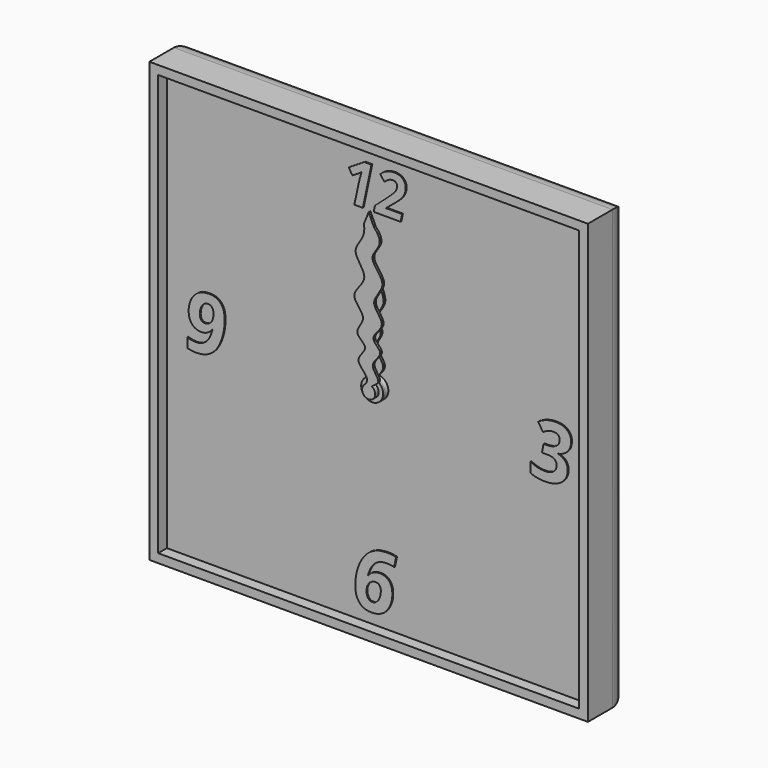
from build123d import *

# Parameters (mm, degrees)
F0_W            = 200
F0_H            = 200
F1_DEPTH        = 24
F2_R            = 10
F3_T            = -4
F4_R            = 5
F4_R_2          = 3
F5_DEPTH        = 2
F6_DEPTH        = 19
F7_DEPTH        = 8
F9_DEPTH        = 4
F11_DEPTH       = 4
F12_R           = 5
F12_R_2         = 3
F13_DEPTH       = 2
F14_R           = 3
F15_DEPTH       = 4
F17_DEPTH       = 4
F18_R           = 3
F19_DEPTH       = 2
F20_W           = 196
F20_H           = 196
F20_R           = 5
F21_DEPTH       = 1
F23_R           = 5
F23_R_2         = 3
F24_DEPTH       = 2
F25_TEXT_SIZE   = 26.048026048
F25_TEXT_SIZE_2 = 34.7222222222
F25_TEXT_SIZE_3 = 35.8387257342
F26_DEPTH       = 0.5
F27_DEPTH       = 1
F28_R           = 5
F28_R_2         = 3
F29_DEPTH       = 5
F30_R           = 3
F31_DEPTH       = 1
F33_DEPTH       = 1
F34_R           = 25
F35_DEPTH       = 10
F36_W           = 1.5
F36_H           = 6
F36_W_2         = 6
F36_H_2         = 1.5
F37_DEPTH       = 0.5
F38_R           = 3.75
F39_DEPTH       = 5
F43_DEPTH       = 1
F45_DEPTH       = 1


# Not quite as in the source:
# - Text() gives the source's letters only with a copy of the font that has no kerning and outlines rounded to 1/6400 em; it was checked with that copy


with BuildPart() as f1:
    # F0 (on Front) → F1 (new body)
    with BuildSketch(Plane.XZ):
        Rectangle(F0_W, F0_H)
    extrude(amount=F1_DEPTH)

    # F2
    f2_edges = [f1.edges().sort_by_distance(p)[0] for p in [
        (0, 0, 100),
        (-100, 0, 0),
        (0, 0, -100),
        (100, 0, 0),
    ]]
    fillet(f2_edges, radius=F2_R)

    # F3
    f3_openings = [f1.faces().sort_by_distance(p)[0] for p in [
        (0, -24, 0),
    ]]
    offset(amount=F3_T, openings=f3_openings)

    # F4 (on face) → F5 (join)
    with BuildSketch(Plane.XZ.offset(4)):
        Circle(F4_R)
        Circle(F4_R_2, mode=Mode.SUBTRACT)
        with Locations((40, 0)):
            Circle(F4_R)
        with Locations((40, 0)):
            Circle(F4_R_2, mode=Mode.SUBTRACT)
    extrude(amount=F5_DEPTH)


with BuildPart() as f6:
    # F6 (new): a face of the model
    f6_faces = [f1.part.faces().sort_by_distance(p)[0] for p in [
        (0, -4, 0),
    ]]
    extrude(f6_faces, amount=F6_DEPTH)

    # F8 (on face) → F9 (join)
    with BuildSketch(Plane.XZ.offset(6)):
        with BuildLine():
            ThreePointArc((9.2729637667, -1.3794085621), (9.3494561423, -0.6915886375), (9.375, 0))
            ThreePointArc((9.375, 0), (9.3494561423, 0.6915886375), (9.2729637667, 1.3794085621))
            ThreePointArc((9.2729637667, 1.3794085621), (8.9161548403, 2.8970343223), (8.3127812852, 4.3345463782))
            ThreePointArc((8.3127812852, 4.3345463782), (7.5845343223, 5.5104867402), (6.6911892658, 6.566476316))
            ThreePointArc((6.6911892658, 6.566476316), (5.5104867402, 7.5845343223), (4.1773988938, 8.3928519278))
            ThreePointArc((4.1773988938, 8.3928519278), (2.8970343223, 8.9161548403), (1.5536078905, 9.2453733036))
            ThreePointArc((1.5536078905, 9.2453733036), (0, 9.375), (-1.5536078905, 9.2453733036))
            ThreePointArc((-1.5536078905, 9.2453733036), (-2.8970343223, 8.9161548403), (-4.1773988938, 8.3928519278))
            ThreePointArc((-4.1773988938, 8.3928519278), (-5.5104867402, 7.5845343223), (-6.6911892658, 6.566476316))
            ThreePointArc((-6.6911892658, 6.566476316), (-7.5845343223, 5.5104867402), (-8.3127812852, 4.3345463782))
            ThreePointArc((-8.3127812852, 4.3345463782), (-8.9161548403, 2.8970343223), (-9.2729637667, 1.3794085621))
            ThreePointArc((-9.2729637667, 1.3794085621), (-9.375, 0), (-9.2729637667, -1.3794085621))
            ThreePointArc((-9.2729637667, -1.3794085621), (-8.9161548403, -2.8970343223), (-8.3127812852, -4.3345463782))
            ThreePointArc((-8.3127812852, -4.3345463782), (-7.5845343223, -5.5104867402), (-6.6911892658, -6.566476316))
            ThreePointArc((-6.6911892658, -6.566476316), (-5.5104867402, -7.5845343223), (-4.1773988938, -8.3928519278))
            ThreePointArc((-4.1773988938, -8.3928519278), (-2.8970343223, -8.9161548403), (-1.5536078905, -9.2453733036))
            ThreePointArc((-1.5536078905, -9.2453733036), (0, -9.375), (1.5536078905, -9.2453733036))
            ThreePointArc((1.5536078905, -9.2453733036), (2.8970343223, -8.9161548403), (4.1773988938, -8.3928519278))
            ThreePointArc((4.1773988938, -8.3928519278), (5.5104867402, -7.5845343223), (6.6911892658, -6.566476316))
            ThreePointArc((6.6911892658, -6.566476316), (7.5845343223, -5.5104867402), (8.3127812852, -4.3345463782))
            ThreePointArc((8.3127812852, -4.3345463782), (8.9161548403, -2.8970343223), (9.2729637667, -1.3794085621))
        make_face()
        with BuildLine():
            ThreePointArc((8.3127812852, 4.3345463782), (8.9161548403, 2.8970343223), (9.2729637667, 1.3794085621))
            Line((9.2729637667, 1.3794085621), (11.1823199426, 2.3946312492))
            Line((11.1823199426, 2.3946312492), (10.8182678729, 3.515068311))
            Line((10.8182678729, 3.515068311), (10.4542158031, 4.6355053728))
            Line((10.4542158031, 4.6355053728), (8.3127812852, 4.3345463782))
        make_face()
        with BuildLine():
            Line((11.1823199426, -2.3946312492), (9.2729637667, -1.3794085621))
            ThreePointArc((9.2729637667, -1.3794085621), (8.9161548403, -2.8970343223), (8.3127812852, -4.3345463782))
            Line((8.3127812852, -4.3345463782), (10.4542158031, -4.6355053728))
            Line((10.4542158031, -4.6355053728), (10.8182678729, -3.515068311))
            Line((10.8182678729, -3.515068311), (11.1823199426, -2.3946312492))
        make_face()
        with BuildLine():
            ThreePointArc((4.1773988938, 8.3928519278), (5.5104867402, 7.5845343223), (6.6911892658, 6.566476316))
            Line((6.6911892658, 6.566476316), (7.6391579371, 8.5101001246))
            Line((7.6391579371, 8.5101001246), (6.6860572448, 9.202568311))
            Line((6.6860572448, 9.202568311), (5.7329565525, 9.8950364974))
            Line((5.7329565525, 9.8950364974), (4.1773988938, 8.3928519278))
        make_face()
        with BuildLine():
            Line((7.6391579371, -8.5101001246), (6.6911892658, -6.566476316))
            ThreePointArc((6.6911892658, -6.566476316), (5.5104867402, -7.5845343223), (4.1773988938, -8.3928519278))
            Line((4.1773988938, -8.3928519278), (5.7329565525, -9.8950364974))
            Line((5.7329565525, -9.8950364974), (6.6860572448, -9.202568311))
            Line((6.6860572448, -9.202568311), (7.6391579371, -8.5101001246))
        make_face()
        with BuildLine():
            ThreePointArc((-1.5536078905, 9.2453733036), (0, 9.375), (1.5536078905, 9.2453733036))
            Line((1.5536078905, 9.2453733036), (1.1780972451, 11.375))
            Line((1.1780972451, 11.375), (0, 11.375))
            Line((0, 11.375), (-1.1780972451, 11.375))
            Line((-1.1780972451, 11.375), (-1.5536078905, 9.2453733036))
        make_face()
        with BuildLine():
            Line((1.1780972451, -11.375), (1.5536078905, -9.2453733036))
            ThreePointArc((1.5536078905, -9.2453733036), (0, -9.375), (-1.5536078905, -9.2453733036))
            Line((-1.5536078905, -9.2453733036), (-1.1780972451, -11.375))
            Line((-1.1780972451, -11.375), (0, -11.375))
            Line((0, -11.375), (1.1780972451, -11.375))
        make_face()
        with BuildLine():
            ThreePointArc((-6.6911892658, 6.566476316), (-5.5104867402, 7.5845343223), (-4.1773988938, 8.3928519278))
            Line((-4.1773988938, 8.3928519278), (-5.7329565525, 9.8950364974))
            Line((-5.7329565525, 9.8950364974), (-6.6860572448, 9.202568311))
            Line((-6.6860572448, 9.202568311), (-7.6391579371, 8.5101001246))
            Line((-7.6391579371, 8.5101001246), (-6.6911892658, 6.566476316))
        make_face()
        with BuildLine():
            Line((-5.7329565525, -9.8950364974), (-4.1773988938, -8.3928519278))
            ThreePointArc((-4.1773988938, -8.3928519278), (-5.5104867402, -7.5845343223), (-6.6911892658, -6.566476316))
            Line((-6.6911892658, -6.566476316), (-7.6391579371, -8.5101001246))
            Line((-7.6391579371, -8.5101001246), (-6.6860572448, -9.202568311))
            Line((-6.6860572448, -9.202568311), (-5.7329565525, -9.8950364974))
        make_face()
        with BuildLine():
            ThreePointArc((-9.2729637667, 1.3794085621), (-8.9161548403, 2.8970343223), (-8.3127812852, 4.3345463782))
            Line((-8.3127812852, 4.3345463782), (-10.4542158031, 4.6355053728))
            Line((-10.4542158031, 4.6355053728), (-10.8182678729, 3.515068311))
            Line((-10.8182678729, 3.515068311), (-11.1823199426, 2.3946312492))
            Line((-11.1823199426, 2.3946312492), (-9.2729637667, 1.3794085621))
        make_face()
        with BuildLine():
            Line((-10.4542158031, -4.6355053728), (-8.3127812852, -4.3345463782))
            ThreePointArc((-8.3127812852, -4.3345463782), (-8.9161548403, -2.8970343223), (-9.2729637667, -1.3794085621))
            Line((-9.2729637667, -1.3794085621), (-11.1823199426, -2.3946312492))
            Line((-11.1823199426, -2.3946312492), (-10.8182678729, -3.515068311))
            Line((-10.8182678729, -3.515068311), (-10.4542158031, -4.6355053728))
        make_face()
    extrude(amount=F9_DEPTH)

    # F32 (on face) → F33 (join)
    with BuildSketch(Plane.XZ.offset(23)):
        with BuildLine():
            ThreePointArc((-1.4071694433, 2.6495045118), (-1.5457185498, -2.5711386903), (3, 0))
            ThreePointArc((3, 0), (2.5711386903, 1.5457185498), (1.4071694433, 2.6495045118))
            ThreePointArc((1.4071694433, 2.6495045118), (0, 3), (-1.4071694433, 2.6495045118))
        make_face()
        with BuildLine():
            ThreePointArc((-1.4071694433, 2.6495045118), (0, 3), (1.4071694433, 2.6495045118))
            add(Edge.make_bspline(
                [(1.4071694433, 2.6495045118), (3.0296074566, 3.8772159389), (6.3039386169, 5.5103249168), (-0.9360700478, 11.6043913935), (8.3069373895, 17.3298364556), (-1.1275149054, 22.1266315872), (9.6827878452, 28.9044203262), (-1.2541438892, 36.5685190657), (10.3089623501, 45.1730816435), (-1.6342219672, 53.9788895131), (6.9529120063, 60.5380152538), (4.0439217419, 65.1597511734), (2.5257738307, 66.6606426239)],
                knots=[0, 0, 0, 0, 0.0782288026, 0.1704201684, 0.2679376052, 0.3576739035, 0.4617977775, 0.5704836043, 0.6853974221, 0.803568051, 0.9061859038, 1, 1, 1, 1], degree=3))
            Line((2.5257738307, 66.6606426239), (0, 72.1388086677))
            Line((0, 72.1388086677), (-2.1966320928, 66.6606426239))
            add(Edge.make_bspline(
                [(-1.4071694433, 2.6495045118), (-0.8303886963, 3.6654317675), (0.0856435734, 6.0391183116), (-7.5716818535, 11.2944408044), (1.3992736808, 17.5147965731), (-8.220861358, 21.8793846794), (0.7776188709, 29.1436053021), (-10.5454136086, 36.5799618446), (2.0038158577, 45.007894694), (-8.7780353011, 54.0426044509), (-2.1019578832, 60.4375853407), (-1.7889988447, 65.0866098847), (-2.1966320928, 66.6606426239)],
                knots=[0, 0, 0, 0, 0.0669744584, 0.165033993, 0.2625239648, 0.3553389335, 0.4570466298, 0.5683341016, 0.6867000587, 0.8048964881, 0.908333357, 1, 1, 1, 1], degree=3))
        make_face()
    extrude(amount=F33_DEPTH)


with BuildPart() as f7:
    # F7 (new): a face of the model
    f7_faces = [f1.part.faces().sort_by_distance(p)[0] for p in [
        (40, -4, 0),
    ]]
    extrude(f7_faces, amount=F7_DEPTH)

    # F10 (on face) → F11 (join)
    with BuildSketch(Plane.XZ.offset(6)):
        with BuildLine():
            ThreePointArc((68.0829066802, -1.5381733945), (68.1144747006, -0.7693746225), (68.125, 0))
            ThreePointArc((68.125, 0), (68.1144747006, 0.7693746225), (68.0829066802, 1.5381733945))
            ThreePointArc((68.0829066802, 1.5381733945), (67.9709283072, 2.9398630294), (67.7890320221, 4.3342039956))
            ThreePointArc((67.7890320221, 4.3342039956), (67.5104012706, 5.8475163042), (67.1494235596, 7.3433252263))
            ThreePointArc((67.1494235596, 7.3433252263), (66.7484645208, 8.6911029668), (66.280643318, 10.0171558733))
            ThreePointArc((66.280643318, 10.0171558733), (65.6934659962, 11.4394680865), (65.0293803521, 12.8275385085))
            ThreePointArc((65.0293803521, 12.8275385085), (64.3569644814, 14.0625), (63.6236643925, 15.2623099717))
            ThreePointArc((63.6236643925, 15.2623099717), (62.7536029668, 16.5314602207), (61.815433119, 17.7511268046))
            ThreePointArc((61.815433119, 17.7511268046), (60.9009482166, 18.8192983038), (59.934217974, 19.8404278876))
            ThreePointArc((59.934217974, 19.8404278876), (58.8192983038, 20.9009482166), (57.6480467764, 21.8989056799))
            ThreePointArc((57.6480467764, 21.8989056799), (56.5314602207, 22.7536029668), (55.3735505752, 23.5514238999))
            ThreePointArc((55.3735505752, 23.5514238999), (54.0625, 24.3569644814), (52.709356105, 25.0895972944))
            ThreePointArc((52.709356105, 25.0895972944), (51.4394680865, 25.6934659962), (50.1409852457, 26.2331096755))
            ThreePointArc((50.1409852457, 26.2331096755), (48.6911029668, 26.7484645208), (47.2152055856, 27.1837531139))
            ThreePointArc((47.2152055856, 27.1837531139), (45.8475163042, 27.5104012706), (44.4652101991, 27.7682826779))
            ThreePointArc((44.4652101991, 27.7682826779), (42.9398630294, 27.9709283072), (41.4057159597, 28.0898484802))
            ThreePointArc((41.4057159597, 28.0898484802), (40, 28.125), (38.5942840403, 28.0898484802))
            ThreePointArc((38.5942840403, 28.0898484802), (37.0601369706, 27.9709283072), (35.5347898009, 27.7682826779))
            ThreePointArc((35.5347898009, 27.7682826779), (34.1524836958, 27.5104012706), (32.7847944144, 27.1837531139))
            ThreePointArc((32.7847944144, 27.1837531139), (31.3088970332, 26.7484645208), (29.8590147543, 26.2331096755))
            ThreePointArc((29.8590147543, 26.2331096755), (28.5605319135, 25.6934659962), (27.290643895, 25.0895972944))
            ThreePointArc((27.290643895, 25.0895972944), (25.9375, 24.3569644814), (24.6264494248, 23.5514238999))
            ThreePointArc((24.6264494248, 23.5514238999), (23.4685397793, 22.7536029668), (22.3519532236, 21.8989056799))
            ThreePointArc((22.3519532236, 21.8989056799), (21.1807016962, 20.9009482166), (20.065782026, 19.8404278876))
            ThreePointArc((20.065782026, 19.8404278876), (19.0990517834, 18.8192983038), (18.184566881, 17.7511268046))
            ThreePointArc((18.184566881, 17.7511268046), (17.2463970332, 16.5314602207), (16.3763356075, 15.2623099717))
            ThreePointArc((16.3763356075, 15.2623099717), (15.6430355186, 14.0625), (14.9706196479, 12.8275385085))
            ThreePointArc((14.9706196479, 12.8275385085), (14.3065340038, 11.4394680865), (13.719356682, 10.0171558733))
            ThreePointArc((13.719356682, 10.0171558733), (13.2515354792, 8.6911029668), (12.8505764404, 7.3433252263))
            ThreePointArc((12.8505764404, 7.3433252263), (12.4895987294, 5.8475163042), (12.2109679779, 4.3342039956))
            ThreePointArc((12.2109679779, 4.3342039956), (12.0290716928, 2.9398630294), (11.9170933198, 1.5381733945))
            ThreePointArc((11.9170933198, 1.5381733945), (11.875, 0), (11.9170933198, -1.5381733945))
            ThreePointArc((11.9170933198, -1.5381733945), (12.0290716928, -2.9398630294), (12.2109679779, -4.3342039956))
            ThreePointArc((12.2109679779, -4.3342039956), (12.4895987294, -5.8475163042), (12.8505764404, -7.3433252263))
            ThreePointArc((12.8505764404, -7.3433252263), (13.2515354792, -8.6911029668), (13.719356682, -10.0171558733))
            ThreePointArc((13.719356682, -10.0171558733), (14.3065340038, -11.4394680865), (14.9706196479, -12.8275385085))
            ThreePointArc((14.9706196479, -12.8275385085), (15.6430355186, -14.0625), (16.3763356075, -15.2623099717))
            ThreePointArc((16.3763356075, -15.2623099717), (17.2463970332, -16.5314602207), (18.184566881, -17.7511268046))
            ThreePointArc((18.184566881, -17.7511268046), (19.0990517834, -18.8192983038), (20.065782026, -19.8404278876))
            ThreePointArc((20.065782026, -19.8404278876), (21.1807016962, -20.9009482166), (22.3519532236, -21.8989056799))
            ThreePointArc((22.3519532236, -21.8989056799), (23.4685397793, -22.7536029668), (24.6264494248, -23.5514238999))
            ThreePointArc((24.6264494248, -23.5514238999), (25.9375, -24.3569644814), (27.290643895, -25.0895972944))
            ThreePointArc((27.290643895, -25.0895972944), (28.5605319135, -25.6934659962), (29.8590147543, -26.2331096755))
            ThreePointArc((29.8590147543, -26.2331096755), (31.3088970332, -26.7484645208), (32.7847944144, -27.1837531139))
            ThreePointArc((32.7847944144, -27.1837531139), (34.1524836958, -27.5104012706), (35.5347898009, -27.7682826779))
            ThreePointArc((35.5347898009, -27.7682826779), (37.0601369706, -27.9709283072), (38.5942840403, -28.0898484802))
            ThreePointArc((38.5942840403, -28.0898484802), (40, -28.125), (41.4057159597, -28.0898484802))
            ThreePointArc((41.4057159597, -28.0898484802), (42.9398630294, -27.9709283072), (44.4652101991, -27.7682826779))
            ThreePointArc((44.4652101991, -27.7682826779), (45.8475163042, -27.5104012706), (47.2152055856, -27.1837531139))
            ThreePointArc((47.2152055856, -27.1837531139), (48.6911029668, -26.7484645208), (50.1409852457, -26.2331096755))
            ThreePointArc((50.1409852457, -26.2331096755), (51.4394680865, -25.6934659962), (52.709356105, -25.0895972944))
            ThreePointArc((52.709356105, -25.0895972944), (54.0625, -24.3569644814), (55.3735505752, -23.5514238999))
            ThreePointArc((55.3735505752, -23.5514238999), (56.5314602207, -22.7536029668), (57.6480467764, -21.8989056799))
            ThreePointArc((57.6480467764, -21.8989056799), (58.8192983038, -20.9009482166), (59.934217974, -19.8404278876))
            ThreePointArc((59.934217974, -19.8404278876), (60.9009482166, -18.8192983038), (61.815433119, -17.7511268046))
            ThreePointArc((61.815433119, -17.7511268046), (62.7536029668, -16.5314602207), (63.6236643925, -15.2623099717))
            ThreePointArc((63.6236643925, -15.2623099717), (64.3569644814, -14.0625), (65.0293803521, -12.8275385085))
            ThreePointArc((65.0293803521, -12.8275385085), (65.6934659962, -11.4394680865), (66.280643318, -10.0171558733))
            ThreePointArc((66.280643318, -10.0171558733), (66.7484645208, -8.6911029668), (67.1494235596, -7.3433252263))
            ThreePointArc((67.1494235596, -7.3433252263), (67.5104012706, -5.8475163042), (67.7890320221, -4.3342039956))
            ThreePointArc((67.7890320221, -4.3342039956), (67.9709283072, -2.9398630294), (68.0829066802, -1.5381733945))
        make_face()
        with BuildLine():
            ThreePointArc((68.0829066802, 1.5381733945), (68.1144747006, 0.7693746225), (68.125, 0))
            ThreePointArc((68.125, 0), (68.1144747006, -0.7693746225), (68.0829066802, -1.5381733945))
            Line((68.0829066802, -1.5381733945), (70.125, -1.1780972451))
            Line((70.125, -1.1780972451), (70.125, 0))
            Line((70.125, 0), (70.125, 1.1780972451))
            Line((70.125, 1.1780972451), (68.0829066802, 1.5381733945))
        make_face()
        with BuildLine():
            ThreePointArc((67.1494235596, 7.3433252263), (67.5104012706, 5.8475163042), (67.7890320221, 4.3342039956))
            Line((67.7890320221, 4.3342039956), (69.7116366623, 5.1109866922))
            Line((69.7116366623, 5.1109866922), (69.4666964721, 6.2633396859))
            Line((69.4666964721, 6.2633396859), (69.2217562819, 7.4156926796))
            Line((69.2217562819, 7.4156926796), (67.1494235596, 7.3433252263))
        make_face()
        with BuildLine():
            Line((69.7116366623, -5.1109866922), (67.7890320221, -4.3342039956))
            ThreePointArc((67.7890320221, -4.3342039956), (67.5104012706, -5.8475163042), (67.1494235596, -7.3433252263))
            Line((67.1494235596, -7.3433252263), (69.2217562819, -7.4156926796))
            Line((69.2217562819, -7.4156926796), (69.4666964721, -6.2633396859))
            Line((69.4666964721, -6.2633396859), (69.7116366623, -5.1109866922))
        make_face()
        with BuildLine():
            ThreePointArc((65.0293803521, 12.8275385085), (65.6934659962, 11.4394680865), (66.280643318, 10.0171558733))
            Line((66.280643318, 10.0171558733), (67.9997322302, 11.1766959857))
            Line((67.9997322302, 11.1766959857), (67.5205569115, 12.2529413727))
            Line((67.5205569115, 12.2529413727), (67.0413815928, 13.3291867596))
            Line((67.0413815928, 13.3291867596), (65.0293803521, 12.8275385085))
        make_face()
        with BuildLine():
            Line((67.9997322302, -11.1766959857), (66.280643318, -10.0171558733))
            ThreePointArc((66.280643318, -10.0171558733), (65.6934659962, -11.4394680865), (65.0293803521, -12.8275385085))
            Line((65.0293803521, -12.8275385085), (67.0413815928, -13.3291867596))
            Line((67.0413815928, -13.3291867596), (67.5205569115, -12.2529413727))
            Line((67.5205569115, -12.2529413727), (67.9997322302, -11.1766959857))
        make_face()
        with BuildLine():
            ThreePointArc((61.815433119, 17.7511268046), (62.7536029668, 16.5314602207), (63.6236643925, 15.2623099717))
            Line((63.6236643925, 15.2623099717), (65.064105142, 16.753930033))
            Line((65.064105142, 16.753930033), (64.3716369555, 17.7070307253))
            Line((64.3716369555, 17.7070307253), (63.6791687691, 18.6601314176))
            Line((63.6791687691, 18.6601314176), (61.815433119, 17.7511268046))
        make_face()
        with BuildLine():
            Line((65.064105142, -16.753930033), (63.6236643925, -15.2623099717))
            ThreePointArc((63.6236643925, -15.2623099717), (62.7536029668, -16.5314602207), (61.815433119, -17.7511268046))
            Line((61.815433119, -17.7511268046), (63.6791687691, -18.6601314176))
            Line((63.6791687691, -18.6601314176), (64.3716369555, -17.7070307253))
            Line((64.3716369555, -17.7070307253), (65.064105142, -16.753930033))
        make_face()
        with BuildLine():
            ThreePointArc((57.6480467764, 21.8989056799), (58.8192983038, 20.9009482166), (59.934217974, 19.8404278876))
            Line((59.934217974, 19.8404278876), (61.0330563882, 21.5989369435))
            Line((61.0330563882, 21.5989369435), (60.1575595166, 22.3872378675))
            Line((60.1575595166, 22.3872378675), (59.282062645, 23.1755387915))
            Line((59.282062645, 23.1755387915), (57.6480467764, 21.8989056799))
        make_face()
        with BuildLine():
            Line((61.0330563882, -21.5989369435), (59.934217974, -19.8404278876))
            ThreePointArc((59.934217974, -19.8404278876), (58.8192983038, -20.9009482166), (57.6480467764, -21.8989056799))
            Line((57.6480467764, -21.8989056799), (59.282062645, -23.1755387915))
            Line((59.282062645, -23.1755387915), (60.1575595166, -22.3872378675))
            Line((60.1575595166, -22.3872378675), (61.0330563882, -21.5989369435))
        make_face()
        with BuildLine():
            ThreePointArc((52.709356105, 25.0895972944), (54.0625, 24.3569644814), (55.3735505752, 23.5514238999))
            Line((55.3735505752, 23.5514238999), (56.0827621424, 25.4999666665))
            Line((56.0827621424, 25.4999666665), (55.0625, 26.089015289))
            Line((55.0625, 26.089015289), (54.0422378576, 26.6780639116))
            Line((54.0422378576, 26.6780639116), (52.709356105, 25.0895972944))
        make_face()
        with BuildLine():
            Line((56.0827621424, -25.4999666665), (55.3735505752, -23.5514238999))
            ThreePointArc((55.3735505752, -23.5514238999), (54.0625, -24.3569644814), (52.709356105, -25.0895972944))
            Line((52.709356105, -25.0895972944), (54.0422378576, -26.6780639116))
            Line((54.0422378576, -26.6780639116), (55.0625, -26.089015289))
            Line((55.0625, -26.089015289), (56.0827621424, -25.4999666665))
        make_face()
        with BuildLine():
            ThreePointArc((47.2152055856, 27.1837531139), (48.6911029668, 26.7484645208), (50.1409852457, 26.2331096755))
            Line((50.1409852457, 26.2331096755), (50.4295740173, 28.2865254836))
            Line((50.4295740173, 28.2865254836), (49.3091369555, 28.6505775534))
            Line((49.3091369555, 28.6505775534), (48.1886998938, 29.0146296232))
            Line((48.1886998938, 29.0146296232), (47.2152055856, 27.1837531139))
        make_face()
        with BuildLine():
            Line((50.4295740173, -28.2865254836), (50.1409852457, -26.2331096755))
            ThreePointArc((50.1409852457, -26.2331096755), (48.6911029668, -26.7484645208), (47.2152055856, -27.1837531139))
            Line((47.2152055856, -27.1837531139), (48.1886998938, -29.0146296232))
            Line((48.1886998938, -29.0146296232), (49.3091369555, -28.6505775534))
            Line((49.3091369555, -28.6505775534), (50.4295740173, -28.2865254836))
        make_face()
        with BuildLine():
            ThreePointArc((41.4057159597, 28.0898484802), (42.9398630294, 27.9709283072), (44.4652101991, 27.7682826779))
            Line((44.4652101991, 27.7682826779), (44.3205634611, 29.8368274034))
            Line((44.3205634611, 29.8368274034), (43.1489199559, 29.959972098))
            Line((43.1489199559, 29.959972098), (41.9772764508, 30.0831167926))
            Line((41.9772764508, 30.0831167926), (41.4057159597, 28.0898484802))
        make_face()
        with BuildLine():
            Line((44.3205634611, -29.8368274034), (44.4652101991, -27.7682826779))
            ThreePointArc((44.4652101991, -27.7682826779), (42.9398630294, -27.9709283072), (41.4057159597, -28.0898484802))
            Line((41.4057159597, -28.0898484802), (41.9772764508, -30.0831167926))
            Line((41.9772764508, -30.0831167926), (43.1489199559, -29.959972098))
            Line((43.1489199559, -29.959972098), (44.3205634611, -29.8368274034))
        make_face()
        with BuildLine():
            ThreePointArc((35.5347898009, 27.7682826779), (37.0601369706, 27.9709283072), (38.5942840403, 28.0898484802))
            Line((38.5942840403, 28.0898484802), (38.0227235492, 30.0831167926))
            Line((38.0227235492, 30.0831167926), (36.8510800441, 29.959972098))
            Line((36.8510800441, 29.959972098), (35.6794365389, 29.8368274034))
            Line((35.6794365389, 29.8368274034), (35.5347898009, 27.7682826779))
        make_face()
        with BuildLine():
            Line((38.0227235492, -30.0831167926), (38.5942840403, -28.0898484802))
            ThreePointArc((38.5942840403, -28.0898484802), (37.0601369706, -27.9709283072), (35.5347898009, -27.7682826779))
            Line((35.5347898009, -27.7682826779), (35.6794365389, -29.8368274034))
            Line((35.6794365389, -29.8368274034), (36.8510800441, -29.959972098))
            Line((36.8510800441, -29.959972098), (38.0227235492, -30.0831167926))
        make_face()
        with BuildLine():
            ThreePointArc((29.8590147543, 26.2331096755), (31.3088970332, 26.7484645208), (32.7847944144, 27.1837531139))
            Line((32.7847944144, 27.1837531139), (31.8113001062, 29.0146296232))
            Line((31.8113001062, 29.0146296232), (30.6908630445, 28.6505775534))
            Line((30.6908630445, 28.6505775534), (29.5704259827, 28.2865254836))
            Line((29.5704259827, 28.2865254836), (29.8590147543, 26.2331096755))
        make_face()
        with BuildLine():
            Line((31.8113001062, -29.0146296232), (32.7847944144, -27.1837531139))
            ThreePointArc((32.7847944144, -27.1837531139), (31.3088970332, -26.7484645208), (29.8590147543, -26.2331096755))
            Line((29.8590147543, -26.2331096755), (29.5704259827, -28.2865254836))
            Line((29.5704259827, -28.2865254836), (30.6908630445, -28.6505775534))
            Line((30.6908630445, -28.6505775534), (31.8113001062, -29.0146296232))
        make_face()
        with BuildLine():
            ThreePointArc((24.6264494248, 23.5514238999), (25.9375, 24.3569644814), (27.290643895, 25.0895972944))
            Line((27.290643895, 25.0895972944), (25.9577621424, 26.6780639116))
            Line((25.9577621424, 26.6780639116), (24.9375, 26.089015289))
            Line((24.9375, 26.089015289), (23.9172378576, 25.4999666665))
            Line((23.9172378576, 25.4999666665), (24.6264494248, 23.5514238999))
        make_face()
        with BuildLine():
            Line((25.9577621424, -26.6780639116), (27.290643895, -25.0895972944))
            ThreePointArc((27.290643895, -25.0895972944), (25.9375, -24.3569644814), (24.6264494248, -23.5514238999))
            Line((24.6264494248, -23.5514238999), (23.9172378576, -25.4999666665))
            Line((23.9172378576, -25.4999666665), (24.9375, -26.089015289))
            Line((24.9375, -26.089015289), (25.9577621424, -26.6780639116))
        make_face()
        with BuildLine():
            ThreePointArc((20.065782026, 19.8404278876), (21.1807016962, 20.9009482166), (22.3519532236, 21.8989056799))
            Line((22.3519532236, 21.8989056799), (20.717937355, 23.1755387915))
            Line((20.717937355, 23.1755387915), (19.8424404834, 22.3872378675))
            Line((19.8424404834, 22.3872378675), (18.9669436118, 21.5989369435))
            Line((18.9669436118, 21.5989369435), (20.065782026, 19.8404278876))
        make_face()
        with BuildLine():
            Line((20.717937355, -23.1755387915), (22.3519532236, -21.8989056799))
            ThreePointArc((22.3519532236, -21.8989056799), (21.1807016962, -20.9009482166), (20.065782026, -19.8404278876))
            Line((20.065782026, -19.8404278876), (18.9669436118, -21.5989369435))
            Line((18.9669436118, -21.5989369435), (19.8424404834, -22.3872378675))
            Line((19.8424404834, -22.3872378675), (20.717937355, -23.1755387915))
        make_face()
        with BuildLine():
            ThreePointArc((16.3763356075, 15.2623099717), (17.2463970332, 16.5314602207), (18.184566881, 17.7511268046))
            Line((18.184566881, 17.7511268046), (16.3208312309, 18.6601314176))
            Line((16.3208312309, 18.6601314176), (15.6283630445, 17.7070307253))
            Line((15.6283630445, 17.7070307253), (14.935894858, 16.753930033))
            Line((14.935894858, 16.753930033), (16.3763356075, 15.2623099717))
        make_face()
        with BuildLine():
            Line((16.3208312309, -18.6601314176), (18.184566881, -17.7511268046))
            ThreePointArc((18.184566881, -17.7511268046), (17.2463970332, -16.5314602207), (16.3763356075, -15.2623099717))
            Line((16.3763356075, -15.2623099717), (14.935894858, -16.753930033))
            Line((14.935894858, -16.753930033), (15.6283630445, -17.7070307253))
            Line((15.6283630445, -17.7070307253), (16.3208312309, -18.6601314176))
        make_face()
        with BuildLine():
            ThreePointArc((13.719356682, 10.0171558733), (14.3065340038, 11.4394680865), (14.9706196479, 12.8275385085))
            Line((14.9706196479, 12.8275385085), (12.9586184072, 13.3291867596))
            Line((12.9586184072, 13.3291867596), (12.4794430885, 12.2529413727))
            Line((12.4794430885, 12.2529413727), (12.0002677698, 11.1766959857))
            Line((12.0002677698, 11.1766959857), (13.719356682, 10.0171558733))
        make_face()
        with BuildLine():
            Line((12.9586184072, -13.3291867596), (14.9706196479, -12.8275385085))
            ThreePointArc((14.9706196479, -12.8275385085), (14.3065340038, -11.4394680865), (13.719356682, -10.0171558733))
            Line((13.719356682, -10.0171558733), (12.0002677698, -11.1766959857))
            Line((12.0002677698, -11.1766959857), (12.4794430885, -12.2529413727))
            Line((12.4794430885, -12.2529413727), (12.9586184072, -13.3291867596))
        make_face()
        with BuildLine():
            ThreePointArc((12.2109679779, 4.3342039956), (12.4895987294, 5.8475163042), (12.8505764404, 7.3433252263))
            Line((12.8505764404, 7.3433252263), (10.7782437181, 7.4156926796))
            Line((10.7782437181, 7.4156926796), (10.5333035279, 6.2633396859))
            Line((10.5333035279, 6.2633396859), (10.2883633377, 5.1109866922))
            Line((10.2883633377, 5.1109866922), (12.2109679779, 4.3342039956))
        make_face()
        with BuildLine():
            Line((10.7782437181, -7.4156926796), (12.8505764404, -7.3433252263))
            ThreePointArc((12.8505764404, -7.3433252263), (12.4895987294, -5.8475163042), (12.2109679779, -4.3342039956))
            Line((12.2109679779, -4.3342039956), (10.2883633377, -5.1109866922))
            Line((10.2883633377, -5.1109866922), (10.5333035279, -6.2633396859))
            Line((10.5333035279, -6.2633396859), (10.7782437181, -7.4156926796))
        make_face()
        with BuildLine():
            ThreePointArc((11.9170933198, -1.5381733945), (11.875, 0), (11.9170933198, 1.5381733945))
            Line((11.9170933198, 1.5381733945), (9.875, 1.1780972451))
            Line((9.875, 1.1780972451), (9.875, 0))
            Line((9.875, 0), (9.875, -1.1780972451))
            Line((9.875, -1.1780972451), (11.9170933198, -1.5381733945))
        make_face()
    extrude(amount=F11_DEPTH)

    # F16 (on face) → F17 (join)
    with BuildSketch(Plane.XZ.offset(12)):
        with BuildLine():
            ThreePointArc((47.4288750323, -1.0304444454), (47.4821976298, -0.5164480894), (47.5, 0))
            ThreePointArc((47.5, 0), (47.4821976298, 0.5164480894), (47.4288750323, 1.0304444454))
            ThreePointArc((47.4288750323, 1.0304444454), (47.1329238722, 2.3176274578), (46.6157661985, 3.532936117))
            ThreePointArc((46.6157661985, 3.532936117), (46.0676274578, 4.4083893922), (45.4044061018, 5.2002302532))
            ThreePointArc((45.4044061018, 5.2002302532), (44.4083893922, 6.0676274578), (43.2756595386, 6.7468551628))
            ThreePointArc((43.2756595386, 6.7468551628), (42.3176274578, 7.1329238722), (41.3156377295, 7.3837048536))
            ThreePointArc((41.3156377295, 7.3837048536), (40, 7.5), (38.6843622705, 7.3837048536))
            ThreePointArc((38.6843622705, 7.3837048536), (37.6823725422, 7.1329238722), (36.7243404614, 6.7468551628))
            ThreePointArc((36.7243404614, 6.7468551628), (35.5916106078, 6.0676274578), (34.5955938982, 5.2002302532))
            ThreePointArc((34.5955938982, 5.2002302532), (33.9323725422, 4.4083893922), (33.3842338015, 3.532936117))
            ThreePointArc((33.3842338015, 3.532936117), (32.8670761278, 2.3176274578), (32.5711249677, 1.0304444454))
            ThreePointArc((32.5711249677, 1.0304444454), (32.5, 0), (32.5711249677, -1.0304444454))
            ThreePointArc((32.5711249677, -1.0304444454), (32.8670761278, -2.3176274578), (33.3842338015, -3.532936117))
            ThreePointArc((33.3842338015, -3.532936117), (33.9323725422, -4.4083893922), (34.5955938982, -5.2002302532))
            ThreePointArc((34.5955938982, -5.2002302532), (35.5916106078, -6.0676274578), (36.7243404614, -6.7468551628))
            ThreePointArc((36.7243404614, -6.7468551628), (37.6823725422, -7.1329238722), (38.6843622705, -7.3837048536))
            ThreePointArc((38.6843622705, -7.3837048536), (40, -7.5), (41.3156377295, -7.3837048536))
            ThreePointArc((41.3156377295, -7.3837048536), (42.3176274578, -7.1329238722), (43.2756595386, -6.7468551628))
            ThreePointArc((43.2756595386, -6.7468551628), (44.4083893922, -6.0676274578), (45.4044061018, -5.2002302532))
            ThreePointArc((45.4044061018, -5.2002302532), (46.0676274578, -4.4083893922), (46.6157661985, -3.532936117))
            ThreePointArc((46.6157661985, -3.532936117), (47.1329238722, -2.3176274578), (47.4288750323, -1.0304444454))
        make_face()
        with BuildLine():
            ThreePointArc((46.6157661985, 3.532936117), (47.1329238722, 2.3176274578), (47.4288750323, 1.0304444454))
            Line((47.4288750323, 1.0304444454), (49.3262785606, 2.0393117971))
            Line((49.3262785606, 2.0393117971), (48.743795249, 3.832011096))
            Line((48.743795249, 3.832011096), (46.6157661985, 3.532936117))
        make_face()
        with BuildLine():
            Line((49.3262785606, -2.0393117971), (47.4288750323, -1.0304444454))
            ThreePointArc((47.4288750323, -1.0304444454), (47.1329238722, -2.3176274578), (46.6157661985, -3.532936117))
            Line((46.6157661985, -3.532936117), (48.743795249, -3.832011096))
            Line((48.743795249, -3.832011096), (49.3262785606, -2.0393117971))
        make_face()
        with BuildLine():
            ThreePointArc((43.2756595386, 6.7468551628), (44.4083893922, 6.0676274578), (45.4044061018, 5.2002302532))
            Line((45.4044061018, 5.2002302532), (46.3464404506, 7.1316868974))
            Line((46.3464404506, 7.1316868974), (44.8214793429, 8.2396359957))
            Line((44.8214793429, 8.2396359957), (43.2756595386, 6.7468551628))
        make_face()
        with BuildLine():
            Line((46.3464404506, -7.1316868974), (45.4044061018, -5.2002302532))
            ThreePointArc((45.4044061018, -5.2002302532), (44.4083893922, -6.0676274578), (43.2756595386, -6.7468551628))
            Line((43.2756595386, -6.7468551628), (44.8214793429, -8.2396359957))
            Line((44.8214793429, -8.2396359957), (46.3464404506, -7.1316868974))
        make_face()
        with BuildLine():
            ThreePointArc((38.6843622705, 7.3837048536), (40, 7.5), (41.3156377295, 7.3837048536))
            Line((41.3156377295, 7.3837048536), (40.9424777961, 9.5))
            Line((40.9424777961, 9.5), (39.0575222039, 9.5))
            Line((39.0575222039, 9.5), (38.6843622705, 7.3837048536))
        make_face()
        with BuildLine():
            Line((40.9424777961, -9.5), (41.3156377295, -7.3837048536))
            ThreePointArc((41.3156377295, -7.3837048536), (40, -7.5), (38.6843622705, -7.3837048536))
            Line((38.6843622705, -7.3837048536), (39.0575222039, -9.5))
            Line((39.0575222039, -9.5), (40.9424777961, -9.5))
        make_face()
        with BuildLine():
            ThreePointArc((34.5955938982, 5.2002302532), (35.5916106078, 6.0676274578), (36.7243404614, 6.7468551628))
            Line((36.7243404614, 6.7468551628), (35.1785206571, 8.2396359957))
            Line((35.1785206571, 8.2396359957), (33.6535595494, 7.1316868974))
            Line((33.6535595494, 7.1316868974), (34.5955938982, 5.2002302532))
        make_face()
        with BuildLine():
            Line((35.1785206571, -8.2396359957), (36.7243404614, -6.7468551628))
            ThreePointArc((36.7243404614, -6.7468551628), (35.5916106078, -6.0676274578), (34.5955938982, -5.2002302532))
            Line((34.5955938982, -5.2002302532), (33.6535595494, -7.1316868974))
            Line((33.6535595494, -7.1316868974), (35.1785206571, -8.2396359957))
        make_face()
        with BuildLine():
            ThreePointArc((32.5711249677, 1.0304444454), (32.8670761278, 2.3176274578), (33.3842338015, 3.532936117))
            Line((33.3842338015, 3.532936117), (31.256204751, 3.832011096))
            Line((31.256204751, 3.832011096), (30.6737214394, 2.0393117971))
            Line((30.6737214394, 2.0393117971), (32.5711249677, 1.0304444454))
        make_face()
        with BuildLine():
            Line((31.256204751, -3.832011096), (33.3842338015, -3.532936117))
            ThreePointArc((33.3842338015, -3.532936117), (32.8670761278, -2.3176274578), (32.5711249677, -1.0304444454))
            Line((32.5711249677, -1.0304444454), (30.6737214394, -2.0393117971))
            Line((30.6737214394, -2.0393117971), (31.256204751, -3.832011096))
        make_face()
    extrude(amount=F17_DEPTH)

    # F18 (on face) → F19 (join)
    with BuildSketch(Plane.XZ.offset(16)):
        with Locations((40, 0)):
            Circle(F18_R)
    extrude(amount=F19_DEPTH)


with BuildPart() as f13:
    # F12 (on face) → F13 (new body)
    with BuildSketch(Plane.XZ.offset(10)):
        Circle(F12_R)
        Circle(F12_R_2, mode=Mode.SUBTRACT)
    extrude(amount=F13_DEPTH)

    # F14 (on face) → F15 (join)
    with BuildSketch(Plane.XZ.offset(12)):
        with BuildLine():
            ThreePointArc((29.9718156995, -1.3001014101), (29.9929530972, -0.6502034357), (30, 0))
            ThreePointArc((30, 0), (29.9929530972, 0.6502034357), (29.9718156995, 1.3001014101))
            ThreePointArc((29.9718156995, 1.3001014101), (29.907520012, 2.3537728718), (29.8061935814, 3.4045299509))
            ThreePointArc((29.8061935814, 3.4045299509), (29.6306502179, 4.6930339512), (29.3994322443, 5.9727199596))
            ThreePointArc((29.3994322443, 5.9727199596), (29.1710976119, 7.0033609157), (28.9066440563, 8.0253304855))
            ThreePointArc((28.9066440563, 8.0253304855), (28.5316954889, 9.2705098312), (28.1031371961, 10.4982703213))
            ThreePointArc((28.1031371961, 10.4982703213), (27.7163859753, 11.480502971), (27.2953170189, 12.448520749))
            ThreePointArc((27.2953170189, 12.448520749), (26.7301957257, 13.6197149922), (26.1148496411, 14.765318426))
            ThreePointArc((26.1148496411, 14.765318426), (25.5792049306, 15.6749569415), (25.0118886885, 16.5651871174))
            ThreePointArc((25.0118886885, 16.5651871174), (24.2705098312, 17.6335575688), (23.4835278178, 18.6687953878))
            ThreePointArc((23.4835278178, 18.6687953878), (22.812178968, 19.4834414499), (22.1125846489, 20.2739636023))
            ThreePointArc((22.1125846489, 20.2739636023), (21.2132034356, 21.2132034356), (20.2739636023, 22.1125846489))
            ThreePointArc((20.2739636023, 22.1125846489), (19.4834414499, 22.812178968), (18.6687953878, 23.4835278178))
            ThreePointArc((18.6687953878, 23.4835278178), (17.6335575688, 24.2705098312), (16.5651871174, 25.0118886885))
            ThreePointArc((16.5651871174, 25.0118886885), (15.6749569415, 25.5792049306), (14.765318426, 26.1148496411))
            ThreePointArc((14.765318426, 26.1148496411), (13.6197149922, 26.7301957257), (12.448520749, 27.2953170189))
            ThreePointArc((12.448520749, 27.2953170189), (11.480502971, 27.7163859753), (10.4982703213, 28.1031371961))
            ThreePointArc((10.4982703213, 28.1031371961), (9.2705098312, 28.5316954889), (8.0253304855, 28.9066440563))
            ThreePointArc((8.0253304855, 28.9066440563), (7.0033609157, 29.1710976119), (5.9727199596, 29.3994322443))
            ThreePointArc((5.9727199596, 29.3994322443), (4.6930339512, 29.6306502179), (3.4045299509, 29.8061935814))
            ThreePointArc((3.4045299509, 29.8061935814), (2.3537728718, 29.907520012), (1.3001014101, 29.9718156995))
            ThreePointArc((1.3001014101, 29.9718156995), (0, 30), (-1.3001014101, 29.9718156995))
            ThreePointArc((-1.3001014101, 29.9718156995), (-2.3537728718, 29.907520012), (-3.4045299509, 29.8061935814))
            ThreePointArc((-3.4045299509, 29.8061935814), (-4.6930339512, 29.6306502179), (-5.9727199596, 29.3994322443))
            ThreePointArc((-5.9727199596, 29.3994322443), (-7.0033609157, 29.1710976119), (-8.0253304855, 28.9066440563))
            ThreePointArc((-8.0253304855, 28.9066440563), (-9.2705098312, 28.5316954889), (-10.4982703213, 28.1031371961))
            ThreePointArc((-10.4982703213, 28.1031371961), (-11.480502971, 27.7163859753), (-12.448520749, 27.2953170189))
            ThreePointArc((-12.448520749, 27.2953170189), (-13.6197149922, 26.7301957257), (-14.765318426, 26.1148496411))
            ThreePointArc((-14.765318426, 26.1148496411), (-15.6749569415, 25.5792049306), (-16.5651871174, 25.0118886885))
            ThreePointArc((-16.5651871174, 25.0118886885), (-17.6335575688, 24.2705098312), (-18.6687953878, 23.4835278178))
            ThreePointArc((-18.6687953878, 23.4835278178), (-19.4834414499, 22.812178968), (-20.2739636023, 22.1125846489))
            ThreePointArc((-20.2739636023, 22.1125846489), (-21.2132034356, 21.2132034356), (-22.1125846489, 20.2739636023))
            ThreePointArc((-22.1125846489, 20.2739636023), (-22.812178968, 19.4834414499), (-23.4835278178, 18.6687953878))
            ThreePointArc((-23.4835278178, 18.6687953878), (-24.2705098312, 17.6335575688), (-25.0118886885, 16.5651871174))
            ThreePointArc((-25.0118886885, 16.5651871174), (-25.5792049306, 15.6749569415), (-26.1148496411, 14.765318426))
            ThreePointArc((-26.1148496411, 14.765318426), (-26.7301957257, 13.6197149922), (-27.2953170189, 12.448520749))
            ThreePointArc((-27.2953170189, 12.448520749), (-27.7163859753, 11.480502971), (-28.1031371961, 10.4982703213))
            ThreePointArc((-28.1031371961, 10.4982703213), (-28.5316954889, 9.2705098312), (-28.9066440563, 8.0253304855))
            ThreePointArc((-28.9066440563, 8.0253304855), (-29.1710976119, 7.0033609157), (-29.3994322443, 5.9727199596))
            ThreePointArc((-29.3994322443, 5.9727199596), (-29.6306502179, 4.6930339512), (-29.8061935814, 3.4045299509))
            ThreePointArc((-29.8061935814, 3.4045299509), (-29.907520012, 2.3537728718), (-29.9718156995, 1.3001014101))
            ThreePointArc((-29.9718156995, 1.3001014101), (-30, 0), (-29.9718156995, -1.3001014101))
            ThreePointArc((-29.9718156995, -1.3001014101), (-29.907520012, -2.3537728718), (-29.8061935814, -3.4045299509))
            ThreePointArc((-29.8061935814, -3.4045299509), (-29.6306502179, -4.6930339512), (-29.3994322443, -5.9727199596))
            ThreePointArc((-29.3994322443, -5.9727199596), (-29.1710976119, -7.0033609157), (-28.9066440563, -8.0253304855))
            ThreePointArc((-28.9066440563, -8.0253304855), (-28.5316954889, -9.2705098312), (-28.1031371961, -10.4982703213))
            ThreePointArc((-28.1031371961, -10.4982703213), (-27.7163859753, -11.480502971), (-27.2953170189, -12.448520749))
            ThreePointArc((-27.2953170189, -12.448520749), (-26.7301957257, -13.6197149922), (-26.1148496411, -14.765318426))
            ThreePointArc((-26.1148496411, -14.765318426), (-25.5792049306, -15.6749569415), (-25.0118886885, -16.5651871174))
            ThreePointArc((-25.0118886885, -16.5651871174), (-24.2705098312, -17.6335575688), (-23.4835278178, -18.6687953878))
            ThreePointArc((-23.4835278178, -18.6687953878), (-22.812178968, -19.4834414499), (-22.1125846489, -20.2739636023))
            ThreePointArc((-22.1125846489, -20.2739636023), (-21.2132034356, -21.2132034356), (-20.2739636023, -22.1125846489))
            ThreePointArc((-20.2739636023, -22.1125846489), (-19.4834414499, -22.812178968), (-18.6687953878, -23.4835278178))
            ThreePointArc((-18.6687953878, -23.4835278178), (-17.6335575688, -24.2705098312), (-16.5651871174, -25.0118886885))
            ThreePointArc((-16.5651871174, -25.0118886885), (-15.6749569415, -25.5792049306), (-14.765318426, -26.1148496411))
            ThreePointArc((-14.765318426, -26.1148496411), (-13.6197149922, -26.7301957257), (-12.448520749, -27.2953170189))
            ThreePointArc((-12.448520749, -27.2953170189), (-11.480502971, -27.7163859753), (-10.4982703213, -28.1031371961))
            ThreePointArc((-10.4982703213, -28.1031371961), (-9.2705098312, -28.5316954889), (-8.0253304855, -28.9066440563))
            ThreePointArc((-8.0253304855, -28.9066440563), (-7.0033609157, -29.1710976119), (-5.9727199596, -29.3994322443))
            ThreePointArc((-5.9727199596, -29.3994322443), (-4.6930339512, -29.6306502179), (-3.4045299509, -29.8061935814))
            ThreePointArc((-3.4045299509, -29.8061935814), (-2.3537728718, -29.907520012), (-1.3001014101, -29.9718156995))
            ThreePointArc((-1.3001014101, -29.9718156995), (0, -30), (1.3001014101, -29.9718156995))
            ThreePointArc((1.3001014101, -29.9718156995), (2.3537728718, -29.907520012), (3.4045299509, -29.8061935814))
            ThreePointArc((3.4045299509, -29.8061935814), (4.6930339512, -29.6306502179), (5.9727199596, -29.3994322443))
            ThreePointArc((5.9727199596, -29.3994322443), (7.0033609157, -29.1710976119), (8.0253304855, -28.9066440563))
            ThreePointArc((8.0253304855, -28.9066440563), (9.2705098312, -28.5316954889), (10.4982703213, -28.1031371961))
            ThreePointArc((10.4982703213, -28.1031371961), (11.480502971, -27.7163859753), (12.448520749, -27.2953170189))
            ThreePointArc((12.448520749, -27.2953170189), (13.6197149922, -26.7301957257), (14.765318426, -26.1148496411))
            ThreePointArc((14.765318426, -26.1148496411), (15.6749569415, -25.5792049306), (16.5651871174, -25.0118886885))
            ThreePointArc((16.5651871174, -25.0118886885), (17.6335575688, -24.2705098312), (18.6687953878, -23.4835278178))
            ThreePointArc((18.6687953878, -23.4835278178), (19.4834414499, -22.812178968), (20.2739636023, -22.1125846489))
            ThreePointArc((20.2739636023, -22.1125846489), (21.2132034356, -21.2132034356), (22.1125846489, -20.2739636023))
            ThreePointArc((22.1125846489, -20.2739636023), (22.812178968, -19.4834414499), (23.4835278178, -18.6687953878))
            ThreePointArc((23.4835278178, -18.6687953878), (24.2705098312, -17.6335575688), (25.0118886885, -16.5651871174))
            ThreePointArc((25.0118886885, -16.5651871174), (25.5792049306, -15.6749569415), (26.1148496411, -14.765318426))
            ThreePointArc((26.1148496411, -14.765318426), (26.7301957257, -13.6197149922), (27.2953170189, -12.448520749))
            ThreePointArc((27.2953170189, -12.448520749), (27.7163859753, -11.480502971), (28.1031371961, -10.4982703213))
            ThreePointArc((28.1031371961, -10.4982703213), (28.5316954889, -9.2705098312), (28.9066440563, -8.0253304855))
            ThreePointArc((28.9066440563, -8.0253304855), (29.1710976119, -7.0033609157), (29.3994322443, -5.9727199596))
            ThreePointArc((29.3994322443, -5.9727199596), (29.6306502179, -4.6930339512), (29.8061935814, -3.4045299509))
            ThreePointArc((29.8061935814, -3.4045299509), (29.907520012, -2.3537728718), (29.9718156995, -1.3001014101))
        make_face()
        Circle(F14_R, mode=Mode.SUBTRACT)
        with BuildLine():
            ThreePointArc((29.9718156995, 1.3001014101), (29.9929530972, 0.6502034357), (30, 0))
            ThreePointArc((30, 0), (29.9929530972, -0.6502034357), (29.9718156995, -1.3001014101))
            Line((29.9718156995, -1.3001014101), (32, -0.9424777961))
            Line((32, -0.9424777961), (32, 0))
            Line((32, 0), (32, 0.9424777961))
            Line((32, 0.9424777961), (29.9718156995, 1.3001014101))
        make_face()
        with BuildLine():
            ThreePointArc((29.3994322443, 5.9727199596), (29.6306502179, 4.6930339512), (29.8061935814, 3.4045299509))
            Line((29.8061935814, 3.4045299509), (31.7534629089, 4.0750285508))
            Line((31.7534629089, 4.0750285508), (31.606026899, 5.0059028813))
            Line((31.606026899, 5.0059028813), (31.4585908892, 5.9367772117))
            Line((31.4585908892, 5.9367772117), (29.3994322443, 5.9727199596))
        make_face()
        with BuildLine():
            Line((31.7534629089, -4.0750285508), (29.8061935814, -3.4045299509))
            ThreePointArc((29.8061935814, -3.4045299509), (29.6306502179, -4.6930339512), (29.3994322443, -5.9727199596))
            Line((29.3994322443, -5.9727199596), (31.4585908892, -5.9367772117))
            Line((31.4585908892, -5.9367772117), (31.606026899, -5.0059028813))
            Line((31.606026899, -5.0059028813), (31.7534629089, -4.0750285508))
        make_face()
        with BuildLine():
            ThreePointArc((28.1031371961, 10.4982703213), (28.5316954889, 9.2705098312), (28.9066440563, 8.0253304855))
            Line((28.9066440563, 8.0253304855), (30.7250501773, 8.9921941706))
            Line((30.7250501773, 8.9921941706), (30.4338085214, 9.88854382))
            Line((30.4338085214, 9.88854382), (30.1425668656, 10.7848934694))
            Line((30.1425668656, 10.7848934694), (28.1031371961, 10.4982703213))
        make_face()
        with BuildLine():
            Line((30.7250501773, -8.9921941706), (28.9066440563, -8.0253304855))
            ThreePointArc((28.9066440563, -8.0253304855), (28.5316954889, -9.2705098312), (28.1031371961, -10.4982703213))
            Line((28.1031371961, -10.4982703213), (30.1425668656, -10.7848934694))
            Line((30.1425668656, -10.7848934694), (30.4338085214, -9.88854382))
            Line((30.4338085214, -9.88854382), (30.7250501773, -8.9921941706))
        make_face()
        with BuildLine():
            ThreePointArc((26.1148496411, 14.765318426), (26.7301957257, 13.6197149922), (27.2953170189, 12.448520749))
            Line((27.2953170189, 12.448520749), (28.9400847397, 13.6879421265))
            Line((28.9400847397, 13.6879421265), (28.512208774, 14.5276959917))
            Line((28.512208774, 14.5276959917), (28.0843328084, 15.3674498569))
            Line((28.0843328084, 15.3674498569), (26.1148496411, 14.765318426))
        make_face()
        with BuildLine():
            Line((28.9400847397, -13.6879421265), (27.2953170189, -12.448520749))
            ThreePointArc((27.2953170189, -12.448520749), (26.7301957257, -13.6197149922), (26.1148496411, -14.765318426))
            Line((26.1148496411, -14.765318426), (28.0843328084, -15.3674498569))
            Line((28.0843328084, -15.3674498569), (28.512208774, -14.5276959917))
            Line((28.512208774, -14.5276959917), (28.9400847397, -13.6879421265))
        make_face()
        with BuildLine():
            ThreePointArc((23.4835278178, 18.6687953878), (24.2705098312, 17.6335575688), (25.0118886885, 16.5651871174))
            Line((25.0118886885, 16.5651871174), (26.4425183691, 18.0466475195))
            Line((26.4425183691, 18.0466475195), (25.88854382, 18.8091280734))
            Line((25.88854382, 18.8091280734), (25.3345692709, 19.5716086272))
            Line((25.3345692709, 19.5716086272), (23.4835278178, 18.6687953878))
        make_face()
        with BuildLine():
            Line((26.4425183691, -18.0466475195), (25.0118886885, -16.5651871174))
            ThreePointArc((25.0118886885, -16.5651871174), (24.2705098312, -17.6335575688), (23.4835278178, -18.6687953878))
            Line((23.4835278178, -18.6687953878), (25.3345692709, -19.5716086272))
            Line((25.3345692709, -19.5716086272), (25.88854382, -18.8091280734))
            Line((25.88854382, -18.8091280734), (26.4425183691, -18.0466475195))
        make_face()
        with BuildLine():
            ThreePointArc((20.2739636023, 22.1125846489), (21.2132034356, 21.2132034356), (22.1125846489, 20.2739636023))
            Line((22.1125846489, 20.2739636023), (23.2938494387, 21.9609845572))
            Line((23.2938494387, 21.9609845572), (22.627416998, 22.627416998))
            Line((22.627416998, 22.627416998), (21.9609845572, 23.2938494387))
            Line((21.9609845572, 23.2938494387), (20.2739636023, 22.1125846489))
        make_face()
        with BuildLine():
            Line((23.2938494387, -21.9609845572), (22.1125846489, -20.2739636023))
            ThreePointArc((22.1125846489, -20.2739636023), (21.2132034356, -21.2132034356), (20.2739636023, -22.1125846489))
            Line((20.2739636023, -22.1125846489), (21.9609845572, -23.2938494387))
            Line((21.9609845572, -23.2938494387), (22.627416998, -22.627416998))
            Line((22.627416998, -22.627416998), (23.2938494387, -21.9609845572))
        make_face()
        with BuildLine():
            ThreePointArc((16.5651871174, 25.0118886885), (17.6335575688, 24.2705098312), (18.6687953878, 23.4835278178))
            Line((18.6687953878, 23.4835278178), (19.5716086272, 25.3345692709))
            Line((19.5716086272, 25.3345692709), (18.8091280734, 25.88854382))
            Line((18.8091280734, 25.88854382), (18.0466475195, 26.4425183691))
            Line((18.0466475195, 26.4425183691), (16.5651871174, 25.0118886885))
        make_face()
        with BuildLine():
            Line((19.5716086272, -25.3345692709), (18.6687953878, -23.4835278178))
            ThreePointArc((18.6687953878, -23.4835278178), (17.6335575688, -24.2705098312), (16.5651871174, -25.0118886885))
            Line((16.5651871174, -25.0118886885), (18.0466475195, -26.4425183691))
            Line((18.0466475195, -26.4425183691), (18.8091280734, -25.88854382))
            Line((18.8091280734, -25.88854382), (19.5716086272, -25.3345692709))
        make_face()
        with BuildLine():
            ThreePointArc((12.448520749, 27.2953170189), (13.6197149922, 26.7301957257), (14.765318426, 26.1148496411))
            Line((14.765318426, 26.1148496411), (15.3674498569, 28.0843328084))
            Line((15.3674498569, 28.0843328084), (14.5276959917, 28.512208774))
            Line((14.5276959917, 28.512208774), (13.6879421265, 28.9400847397))
            Line((13.6879421265, 28.9400847397), (12.448520749, 27.2953170189))
        make_face()
        with BuildLine():
            Line((15.3674498569, -28.0843328084), (14.765318426, -26.1148496411))
            ThreePointArc((14.765318426, -26.1148496411), (13.6197149922, -26.7301957257), (12.448520749, -27.2953170189))
            Line((12.448520749, -27.2953170189), (13.6879421265, -28.9400847397))
            Line((13.6879421265, -28.9400847397), (14.5276959917, -28.512208774))
            Line((14.5276959917, -28.512208774), (15.3674498569, -28.0843328084))
        make_face()
        with BuildLine():
            ThreePointArc((8.0253304855, 28.9066440563), (9.2705098312, 28.5316954889), (10.4982703213, 28.1031371961))
            Line((10.4982703213, 28.1031371961), (10.7848934694, 30.1425668656))
            Line((10.7848934694, 30.1425668656), (9.88854382, 30.4338085214))
            Line((9.88854382, 30.4338085214), (8.9921941706, 30.7250501773))
            Line((8.9921941706, 30.7250501773), (8.0253304855, 28.9066440563))
        make_face()
        with BuildLine():
            Line((10.7848934694, -30.1425668656), (10.4982703213, -28.1031371961))
            ThreePointArc((10.4982703213, -28.1031371961), (9.2705098312, -28.5316954889), (8.0253304855, -28.9066440563))
            Line((8.0253304855, -28.9066440563), (8.9921941706, -30.7250501773))
            Line((8.9921941706, -30.7250501773), (9.88854382, -30.4338085214))
            Line((9.88854382, -30.4338085214), (10.7848934694, -30.1425668656))
        make_face()
        with BuildLine():
            ThreePointArc((3.4045299509, 29.8061935814), (4.6930339512, 29.6306502179), (5.9727199596, 29.3994322443))
            Line((5.9727199596, 29.3994322443), (5.9367772117, 31.4585908892))
            Line((5.9367772117, 31.4585908892), (5.0059028813, 31.606026899))
            Line((5.0059028813, 31.606026899), (4.0750285508, 31.7534629089))
            Line((4.0750285508, 31.7534629089), (3.4045299509, 29.8061935814))
        make_face()
        with BuildLine():
            Line((5.9367772117, -31.4585908892), (5.9727199596, -29.3994322443))
            ThreePointArc((5.9727199596, -29.3994322443), (4.6930339512, -29.6306502179), (3.4045299509, -29.8061935814))
            Line((3.4045299509, -29.8061935814), (4.0750285508, -31.7534629089))
            Line((4.0750285508, -31.7534629089), (5.0059028813, -31.606026899))
            Line((5.0059028813, -31.606026899), (5.9367772117, -31.4585908892))
        make_face()
        with BuildLine():
            ThreePointArc((-1.3001014101, 29.9718156995), (0, 30), (1.3001014101, 29.9718156995))
            Line((1.3001014101, 29.9718156995), (0.9424777961, 32))
            Line((0.9424777961, 32), (0, 32))
            Line((0, 32), (-0.9424777961, 32))
            Line((-0.9424777961, 32), (-1.3001014101, 29.9718156995))
        make_face()
        with BuildLine():
            Line((0.9424777961, -32), (1.3001014101, -29.9718156995))
            ThreePointArc((1.3001014101, -29.9718156995), (0, -30), (-1.3001014101, -29.9718156995))
            Line((-1.3001014101, -29.9718156995), (-0.9424777961, -32))
            Line((-0.9424777961, -32), (0, -32))
            Line((0, -32), (0.9424777961, -32))
        make_face()
        with BuildLine():
            ThreePointArc((-5.9727199596, 29.3994322443), (-4.6930339512, 29.6306502179), (-3.4045299509, 29.8061935814))
            Line((-3.4045299509, 29.8061935814), (-4.0750285508, 31.7534629089))
            Line((-4.0750285508, 31.7534629089), (-5.0059028813, 31.606026899))
            Line((-5.0059028813, 31.606026899), (-5.9367772117, 31.4585908892))
            Line((-5.9367772117, 31.4585908892), (-5.9727199596, 29.3994322443))
        make_face()
        with BuildLine():
            Line((-4.0750285508, -31.7534629089), (-3.4045299509, -29.8061935814))
            ThreePointArc((-3.4045299509, -29.8061935814), (-4.6930339512, -29.6306502179), (-5.9727199596, -29.3994322443))
            Line((-5.9727199596, -29.3994322443), (-5.9367772117, -31.4585908892))
            Line((-5.9367772117, -31.4585908892), (-5.0059028813, -31.606026899))
            Line((-5.0059028813, -31.606026899), (-4.0750285508, -31.7534629089))
        make_face()
        with BuildLine():
            ThreePointArc((-10.4982703213, 28.1031371961), (-9.2705098312, 28.5316954889), (-8.0253304855, 28.9066440563))
            Line((-8.0253304855, 28.9066440563), (-8.9921941706, 30.7250501773))
            Line((-8.9921941706, 30.7250501773), (-9.88854382, 30.4338085214))
            Line((-9.88854382, 30.4338085214), (-10.7848934694, 30.1425668656))
            Line((-10.7848934694, 30.1425668656), (-10.4982703213, 28.1031371961))
        make_face()
        with BuildLine():
            Line((-8.9921941706, -30.7250501773), (-8.0253304855, -28.9066440563))
            ThreePointArc((-8.0253304855, -28.9066440563), (-9.2705098312, -28.5316954889), (-10.4982703213, -28.1031371961))
            Line((-10.4982703213, -28.1031371961), (-10.7848934694, -30.1425668656))
            Line((-10.7848934694, -30.1425668656), (-9.88854382, -30.4338085214))
            Line((-9.88854382, -30.4338085214), (-8.9921941706, -30.7250501773))
        make_face()
        with BuildLine():
            ThreePointArc((-14.765318426, 26.1148496411), (-13.6197149922, 26.7301957257), (-12.448520749, 27.2953170189))
            Line((-12.448520749, 27.2953170189), (-13.6879421265, 28.9400847397))
            Line((-13.6879421265, 28.9400847397), (-14.5276959917, 28.512208774))
            Line((-14.5276959917, 28.512208774), (-15.3674498569, 28.0843328084))
            Line((-15.3674498569, 28.0843328084), (-14.765318426, 26.1148496411))
        make_face()
        with BuildLine():
            Line((-13.6879421265, -28.9400847397), (-12.448520749, -27.2953170189))
            ThreePointArc((-12.448520749, -27.2953170189), (-13.6197149922, -26.7301957257), (-14.765318426, -26.1148496411))
            Line((-14.765318426, -26.1148496411), (-15.3674498569, -28.0843328084))
            Line((-15.3674498569, -28.0843328084), (-14.5276959917, -28.512208774))
            Line((-14.5276959917, -28.512208774), (-13.6879421265, -28.9400847397))
        make_face()
        with BuildLine():
            ThreePointArc((-18.6687953878, 23.4835278178), (-17.6335575688, 24.2705098312), (-16.5651871174, 25.0118886885))
            Line((-16.5651871174, 25.0118886885), (-18.0466475195, 26.4425183691))
            Line((-18.0466475195, 26.4425183691), (-18.8091280734, 25.88854382))
            Line((-18.8091280734, 25.88854382), (-19.5716086272, 25.3345692709))
            Line((-19.5716086272, 25.3345692709), (-18.6687953878, 23.4835278178))
        make_face()
        with BuildLine():
            Line((-18.0466475195, -26.4425183691), (-16.5651871174, -25.0118886885))
            ThreePointArc((-16.5651871174, -25.0118886885), (-17.6335575688, -24.2705098312), (-18.6687953878, -23.4835278178))
            Line((-18.6687953878, -23.4835278178), (-19.5716086272, -25.3345692709))
            Line((-19.5716086272, -25.3345692709), (-18.8091280734, -25.88854382))
            Line((-18.8091280734, -25.88854382), (-18.0466475195, -26.4425183691))
        make_face()
        with BuildLine():
            ThreePointArc((-22.1125846489, 20.2739636023), (-21.2132034356, 21.2132034356), (-20.2739636023, 22.1125846489))
            Line((-20.2739636023, 22.1125846489), (-21.9609845572, 23.2938494387))
            Line((-21.9609845572, 23.2938494387), (-22.627416998, 22.627416998))
            Line((-22.627416998, 22.627416998), (-23.2938494387, 21.9609845572))
            Line((-23.2938494387, 21.9609845572), (-22.1125846489, 20.2739636023))
        make_face()
        with BuildLine():
            Line((-21.9609845572, -23.2938494387), (-20.2739636023, -22.1125846489))
            ThreePointArc((-20.2739636023, -22.1125846489), (-21.2132034356, -21.2132034356), (-22.1125846489, -20.2739636023))
            Line((-22.1125846489, -20.2739636023), (-23.2938494387, -21.9609845572))
            Line((-23.2938494387, -21.9609845572), (-22.627416998, -22.627416998))
            Line((-22.627416998, -22.627416998), (-21.9609845572, -23.2938494387))
        make_face()
        with BuildLine():
            ThreePointArc((-25.0118886885, 16.5651871174), (-24.2705098312, 17.6335575688), (-23.4835278178, 18.6687953878))
            Line((-23.4835278178, 18.6687953878), (-25.3345692709, 19.5716086272))
            Line((-25.3345692709, 19.5716086272), (-25.88854382, 18.8091280734))
            Line((-25.88854382, 18.8091280734), (-26.4425183691, 18.0466475195))
            Line((-26.4425183691, 18.0466475195), (-25.0118886885, 16.5651871174))
        make_face()
        with BuildLine():
            Line((-25.3345692709, -19.5716086272), (-23.4835278178, -18.6687953878))
            ThreePointArc((-23.4835278178, -18.6687953878), (-24.2705098312, -17.6335575688), (-25.0118886885, -16.5651871174))
            Line((-25.0118886885, -16.5651871174), (-26.4425183691, -18.0466475195))
            Line((-26.4425183691, -18.0466475195), (-25.88854382, -18.8091280734))
            Line((-25.88854382, -18.8091280734), (-25.3345692709, -19.5716086272))
        make_face()
        with BuildLine():
            ThreePointArc((-27.2953170189, 12.448520749), (-26.7301957257, 13.6197149922), (-26.1148496411, 14.765318426))
            Line((-26.1148496411, 14.765318426), (-28.0843328084, 15.3674498569))
            Line((-28.0843328084, 15.3674498569), (-28.512208774, 14.5276959917))
            Line((-28.512208774, 14.5276959917), (-28.9400847397, 13.6879421265))
            Line((-28.9400847397, 13.6879421265), (-27.2953170189, 12.448520749))
        make_face()
        with BuildLine():
            Line((-28.0843328084, -15.3674498569), (-26.1148496411, -14.765318426))
            ThreePointArc((-26.1148496411, -14.765318426), (-26.7301957257, -13.6197149922), (-27.2953170189, -12.448520749))
            Line((-27.2953170189, -12.448520749), (-28.9400847397, -13.6879421265))
            Line((-28.9400847397, -13.6879421265), (-28.512208774, -14.5276959917))
            Line((-28.512208774, -14.5276959917), (-28.0843328084, -15.3674498569))
        make_face()
        with BuildLine():
            ThreePointArc((-28.9066440563, 8.0253304855), (-28.5316954889, 9.2705098312), (-28.1031371961, 10.4982703213))
            Line((-28.1031371961, 10.4982703213), (-30.1425668656, 10.7848934694))
            Line((-30.1425668656, 10.7848934694), (-30.4338085214, 9.88854382))
            Line((-30.4338085214, 9.88854382), (-30.7250501773, 8.9921941706))
            Line((-30.7250501773, 8.9921941706), (-28.9066440563, 8.0253304855))
        make_face()
        with BuildLine():
            Line((-30.1425668656, -10.7848934694), (-28.1031371961, -10.4982703213))
            ThreePointArc((-28.1031371961, -10.4982703213), (-28.5316954889, -9.2705098312), (-28.9066440563, -8.0253304855))
            Line((-28.9066440563, -8.0253304855), (-30.7250501773, -8.9921941706))
            Line((-30.7250501773, -8.9921941706), (-30.4338085214, -9.88854382))
            Line((-30.4338085214, -9.88854382), (-30.1425668656, -10.7848934694))
        make_face()
        with BuildLine():
            ThreePointArc((-29.8061935814, 3.4045299509), (-29.6306502179, 4.6930339512), (-29.3994322443, 5.9727199596))
            Line((-29.3994322443, 5.9727199596), (-31.4585908892, 5.9367772117))
            Line((-31.4585908892, 5.9367772117), (-31.606026899, 5.0059028813))
            Line((-31.606026899, 5.0059028813), (-31.7534629089, 4.0750285508))
            Line((-31.7534629089, 4.0750285508), (-29.8061935814, 3.4045299509))
        make_face()
        with BuildLine():
            Line((-31.4585908892, -5.9367772117), (-29.3994322443, -5.9727199596))
            ThreePointArc((-29.3994322443, -5.9727199596), (-29.6306502179, -4.6930339512), (-29.8061935814, -3.4045299509))
            Line((-29.8061935814, -3.4045299509), (-31.7534629089, -4.0750285508))
            Line((-31.7534629089, -4.0750285508), (-31.606026899, -5.0059028813))
            Line((-31.606026899, -5.0059028813), (-31.4585908892, -5.9367772117))
        make_face()
        with BuildLine():
            ThreePointArc((-29.9718156995, -1.3001014101), (-30, 0), (-29.9718156995, 1.3001014101))
            Line((-29.9718156995, 1.3001014101), (-32, 0.9424777961))
            Line((-32, 0.9424777961), (-32, 0))
            Line((-32, 0), (-32, -0.9424777961))
            Line((-32, -0.9424777961), (-29.9718156995, -1.3001014101))
        make_face()
    extrude(amount=F15_DEPTH)

    # F28 (on face) → F29 (join)
    with BuildSketch(Plane.XZ.offset(16)):
        Circle(F28_R)
        Circle(F28_R_2, mode=Mode.SUBTRACT)
    extrude(amount=F29_DEPTH)

    # F30 (on face) → F31 (join)
    with BuildSketch(Plane.XZ.offset(21)):
        with BuildLine():
            ThreePointArc((-1.070723664, 4.8840097088), (-3.1341970008, -3.8957424401), (5, 0))
            ThreePointArc((5, 0), (3.8957424401, 3.1341970008), (1.070723664, 4.8840097088))
            ThreePointArc((1.070723664, 4.8840097088), (0, 5), (-1.070723664, 4.8840097088))
        make_face()
        Circle(F30_R, mode=Mode.SUBTRACT)
        with BuildLine():
            ThreePointArc((-1.070723664, 4.8840097088), (0, 5), (1.070723664, 4.8840097088))
            add(Edge.make_bspline(
                [(1.070723664, 4.8840097088), (2.1314861839, 6.2959193276), (8.128105866, 10.9072243346), (-1.3345187153, 17.4392756527), (6.2502784862, 23.9344176885), (-0.7140044356, 29.7938822126), (8.7980041153, 36.6104852087), (1.2816021581, 45.9442712417), (0, 48.258561641)],
                knots=[0, 0, 0, 0, 0.1580136082, 0.3223325595, 0.4768667611, 0.6213357646, 0.7909726933, 1, 1, 1, 1], degree=3))
            add(Edge.make_bspline(
                [(-1.070723664, 4.8840097088), (-2.1314861839, 6.2959193276), (-8.128105866, 10.9072243346), (1.3345187153, 17.4392756527), (-6.2502784862, 23.9344176885), (0.7140044356, 29.7938822126), (-8.7980041153, 36.6104852087), (-1.2816021581, 45.9442712417), (0, 48.258561641)],
                knots=[0, 0, 0, 0, 0.1580136082, 0.3223325595, 0.4768667611, 0.6213357646, 0.7909726933, 1, 1, 1, 1], degree=3))
        make_face()
    extrude(amount=F31_DEPTH)


with BuildPart() as f21:
    # F20 (on face) → F21 (new body)
    with BuildSketch(Plane.XZ.offset(18)):
        Rectangle(F20_W, F20_H)
        Circle(F20_R, mode=Mode.SUBTRACT)
    extrude(amount=F21_DEPTH)


with BuildPart() as f1_1:
    add(f1.part)

    # F22: cut F21
    add(f21.part, mode=Mode.SUBTRACT)

    # F34 (on face) → F35 (join)
    with BuildSketch(Plane(origin=(0, 0, 0), x_dir=(-1, 0, 0), z_dir=(0, 1, 0))):
        Circle(F34_R)
    extrude(amount=F35_DEPTH)

    # F36 (on face) → F37 (cut)
    with BuildSketch(Plane(origin=(0, 10, 0), x_dir=(-1, 0, 0), z_dir=(0, 1, 0))):
        with Locations((0, 20)):
            Rectangle(F36_W, F36_H)
        Polygon((-10.8504809472, 20.293584287), (-12.1495190528, 19.543584287), (-9.1495190528, 14.3474318643), (-7.8504809472, 15.0974318643), align=None)
        Polygon((-19.543584287, 12.1495190528), (-20.293584287, 10.8504809472), (-15.0974318643, 7.8504809472), (-14.3474318643, 9.1495190528), align=None)
        with Locations((-20, 0)):
            Rectangle(F36_W_2, F36_H_2)
        Polygon((-20.293584287, -10.8504809472), (-19.543584287, -12.1495190528), (-14.3474318643, -9.1495190528), (-15.0974318643, -7.8504809472), align=None)
        Polygon((-12.1495190528, -19.543584287), (-10.8504809472, -20.293584287), (-7.8504809472, -15.0974318643), (-9.1495190528, -14.3474318643), align=None)
        with Locations((0, -20)):
            Rectangle(F36_W, F36_H)
        Polygon((10.8504809472, -20.293584287), (12.1495190528, -19.543584287), (9.1495190528, -14.3474318643), (7.8504809472, -15.0974318643), align=None)
        Polygon((19.543584287, -12.1495190528), (20.293584287, -10.8504809472), (15.0974318643, -7.8504809472), (14.3474318643, -9.1495190528), align=None)
        with Locations((20, 0)):
            Rectangle(F36_W_2, F36_H_2)
        Polygon((20.293584287, 10.8504809472), (19.543584287, 12.1495190528), (14.3474318643, 9.1495190528), (15.0974318643, 7.8504809472), align=None)
        Polygon((12.1495190528, 19.543584287), (10.8504809472, 20.293584287), (7.8504809472, 15.0974318643), (9.1495190528, 14.3474318643), align=None)
    extrude(amount=-F37_DEPTH, mode=Mode.SUBTRACT)


with BuildPart() as f21_1:
    add(f21.part)

    # F23 (on face) → F24 (join, through all)
    with BuildSketch(Plane(origin=(0, -18, 0), x_dir=(-1, 0, 0), z_dir=(0, 1, 0))):
        with Locations((-40, 0)):
            Circle(F23_R)
        with Locations((-40, 0)):
            Circle(F23_R_2, mode=Mode.SUBTRACT)
    extrude(amount=F24_DEPTH)

    # F25 (on face) → F26 (cut)
    with BuildSketch(Plane.XZ.offset(19)):
        with Locations((-15, 70)):
            Text('12', F25_TEXT_SIZE, font='Open Sans', font_style=FontStyle.BOLDITALIC, text_align=(TextAlign.LEFT, TextAlign.BOTTOM))
        with Locations((70, -12.5)):
            Text('3', F25_TEXT_SIZE_2, font='Open Sans', font_style=FontStyle.BOLDITALIC, text_align=(TextAlign.LEFT, TextAlign.BOTTOM))
        with Locations((-11.25, -90.8038825286)):
            Text('6', F25_TEXT_SIZE_3, font='Open Sans', font_style=FontStyle.BOLDITALIC, text_align=(TextAlign.LEFT, TextAlign.BOTTOM))
        with Locations((-87.7682291667, -12.5)):
            Text('9', F25_TEXT_SIZE_2, font='Open Sans', font_style=FontStyle.BOLDITALIC, text_align=(TextAlign.LEFT, TextAlign.BOTTOM))
    extrude(amount=-F26_DEPTH, mode=Mode.SUBTRACT)


with BuildPart() as f27:
    # F27 (new): a face of the model
    f27_faces = [f21_1.part.faces().sort_by_distance(p)[0] for p in [
        (-6.8641928221, -18.5, 80.3713515652),
    ]]
    extrude(f27_faces, amount=F27_DEPTH)


with BuildPart() as f27b:
    # F27#2 (new): a face of the model
    f27_2_faces = [f21_1.part.faces().sort_by_distance(p)[0] for p in [
        (6.9224467406, -18.5, 78.7533704119),
    ]]
    extrude(f27_2_faces, amount=F27_DEPTH)


with BuildPart() as f27c:
    # F27#3 (new): a face of the model
    f27_3_faces = [f21_1.part.faces().sort_by_distance(p)[0] for p in [
        (81.0972677263, -18.5, -0.3445018213),
    ]]
    extrude(f27_3_faces, amount=F27_DEPTH)


with BuildPart() as f27d:
    # F27#4 (new): a face of the model
    f27_4_faces = [f21_1.part.faces().sort_by_distance(p)[0] for p in [
        (-7.0008137235, -18.5, -89.3066111769),
    ]]
    extrude(f27_4_faces, amount=F27_DEPTH)


with BuildPart() as f27e:
    # F27#5 (new): a face of the model
    f27_5_faces = [f21_1.part.faces().sort_by_distance(p)[0] for p in [
        (-71.990432084, -18.5, 11.084211076),
    ]]
    extrude(f27_5_faces, amount=F27_DEPTH)


with BuildPart() as f39:
    # F38 (on face) → F39 (new body, symmetric)
    with BuildSketch(Plane(origin=(0, 10, 0), x_dir=(-1, 0, 0), z_dir=(0, 1, 0))):
        Circle(F38_R)
    extrude(amount=F39_DEPTH, both=True)


with BuildPart() as f1_2:
    add(f1_1.part)

    # F40: cut F39
    add(f39.part, mode=Mode.SUBTRACT)


with BuildPart() as f39_1:
    add(f39.part)

    # F42 (on offset) → F43 (cut)
    with BuildSketch(Plane(origin=(0, 13, 0), x_dir=(-1, 0, 0), z_dir=(0, 1, 0))):
        Polygon((-0.5, 7.0635083269), (-0.5, 3.3135083269), (0, 3.3135083269), (0.5, 3.3135083269), (0.5, 7.0635083269), (0, 9), align=None)
        Polygon((-1.9476313279, 2.6806845475), (-1.5431228307, 2.9745771736), (-3.7473175268, 6.0083909025), (-5.2900672706, 7.2811529494), (-4.5563345212, 5.4206056502), (-2.3521398251, 2.3867919213), align=None)
        Polygon((-3.1513336861, 1.023930384), (-2.9968251889, 1.4994586422), (-6.563287125, 2.6582723711), (-8.5595086467, 2.7811529494), (-6.8723041194, 1.7072158548), (-3.3058421833, 0.5484021259), align=None)
        Polygon((-3.1513336861, -1.023930384), (-3.3058421833, -0.5484021259), (-6.8723041194, -1.7072158548), (-8.5595086467, -2.7811529494), (-6.563287125, -2.6582723711), (-2.9968251889, -1.4994586422), align=None)
        Polygon((-1.9476313279, -2.6806845475), (-2.3521398251, -2.3867919213), (-4.5563345212, -5.4206056502), (-5.2900672706, -7.2811529494), (-3.7473175268, -6.0083909025), (-1.5431228307, -2.9745771736), align=None)
        Polygon((0, -3.3135083269), (-0.5, -3.3135083269), (-0.5, -7.0635083269), (0, -9), (0.5, -7.0635083269), (0.5, -3.3135083269), align=None)
        Polygon((1.9476313279, -2.6806845475), (1.5431228307, -2.9745771736), (3.7473175268, -6.0083909025), (5.2900672706, -7.2811529494), (4.5563345212, -5.4206056502), (2.3521398251, -2.3867919213), align=None)
        Polygon((3.1513336861, -1.023930384), (2.9968251889, -1.4994586422), (6.563287125, -2.6582723711), (8.5595086467, -2.7811529494), (6.8723041194, -1.7072158548), (3.3058421833, -0.5484021259), align=None)
        Polygon((3.1513336861, 1.023930384), (3.3058421833, 0.5484021259), (6.8723041194, 1.7072158548), (8.5595086467, 2.7811529494), (6.563287125, 2.6582723711), (2.9968251889, 1.4994586422), align=None)
        Polygon((1.9476313279, 2.6806845475), (2.3521398251, 2.3867919213), (4.5563345212, 5.4206056502), (5.2900672706, 7.2811529494), (3.7473175268, 6.0083909025), (1.5431228307, 2.9745771736), align=None)
    extrude(amount=-F43_DEPTH, mode=Mode.SUBTRACT)


with BuildPart() as f45:
    # F44 (on offset) → F45 (new body)
    with BuildSketch(Plane(origin=(0, 13, 0), x_dir=(-1, 0, 0), z_dir=(0, 1, 0))):
        Polygon((-0.5, 7.0635083269), (-0.5, 3.3135083269), (0, 3.3135083269), (0.5, 3.3135083269), (0.5, 7.0635083269), (0, 9), align=None)
    extrude(amount=-F45_DEPTH)


solid = Compound([f6.part, f7.part, f13.part, f21_1.part, f27.part, f27b.part, f27c.part, f27d.part, f27e.part, f1_2.part, f39_1.part, f45.part])
